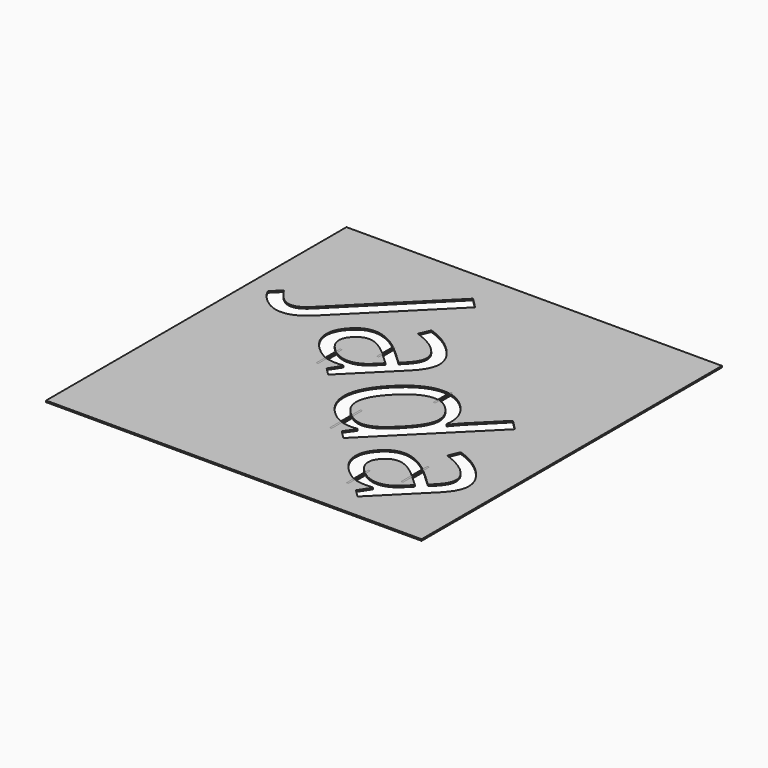
from build123d import *

# Parameters (mm, degrees)
F0_W         = 100
F0_H         = 100
F1_DEPTH     = 0.4
F2_TEXT_SIZE = 47.2500001908
F3_DEPTH     = 25
F4_W         = 0.5
F4_H         = 5.3818935527
F5_DEPTH     = 0.4
F4_H_2       = 5.7719018951
F4_H_3       = 8.7648686022
F4_H_4       = 7.9566752538
F4_H_5       = 10.2641098201
F4_H_6       = 7.2405748069


# Not quite as in the source:
# - Text() gives the source's letters only with a copy of the font that has no kerning and outlines rounded to 1/6400 em; it was checked with that copy


with BuildPart() as f1:
    # F0 (on Top) → F1 (new body)
    with BuildSketch(Plane.XY):
        Rectangle(F0_W, F0_H)
    extrude(amount=F1_DEPTH)

    # F2 (on face) → F3 (cut)
    with BuildSketch(Plane.XY.offset(0.4)):
        with Locations(Location((-36.2654561258, 20.5326806586), (0, 0, -45))):
            Text('Jada', F2_TEXT_SIZE, font='Open Sans', text_align=(TextAlign.LEFT, TextAlign.BOTTOM))
    extrude(amount=-F3_DEPTH, mode=Mode.SUBTRACT)


with BuildPart() as f5:
    # F4 (on Top) → F5 (new body)
    with BuildSketch(Plane.XY):
        with Locations((-8.4556083039, 11.2270636592)):
            Rectangle(F4_W, F4_H)
    extrude(amount=F5_DEPTH)


with BuildPart() as f5b:
    # F4 (on Top) → F5, piece 2 (new body)
    with BuildSketch(Plane.XY):
        with Locations((13.6451073512, 2.5417085417)):
            Rectangle(F4_W, F4_H_2)
    extrude(amount=F5_DEPTH)


with BuildPart() as f5c:
    # F4 (on Top) → F5, piece 3 (new body)
    with BuildSketch(Plane.XY):
        with Locations((30.716299504, -27.9963547364)):
            Rectangle(F4_W, F4_H_3)
    extrude(amount=F5_DEPTH)


with BuildPart() as f5d:
    # F4 (on Top) → F5, piece 4 (new body)
    with BuildSketch(Plane.XY):
        with Locations((-16.4819346219, 2.3580244742)):
            Rectangle(F4_W, F4_H_4)
    extrude(amount=F5_DEPTH)


with BuildPart() as f5e:
    # F4 (on Top) → F5, piece 5 (new body)
    with BuildSketch(Plane.XY):
        with Locations((3.9667188711, -17.5734460354)):
            Rectangle(F4_W, F4_H_5)
    extrude(amount=F5_DEPTH)


with BuildPart() as f5f:
    # F4 (on Top) → F5, piece 6 (new body)
    with BuildSketch(Plane.XY):
        with Locations((22.1875044107, -36.271629855)):
            Rectangle(F4_W, F4_H_6)
    extrude(amount=F5_DEPTH)


solid = Compound([f1.part, f5.part, f5b.part, f5c.part, f5d.part, f5e.part, f5f.part])
